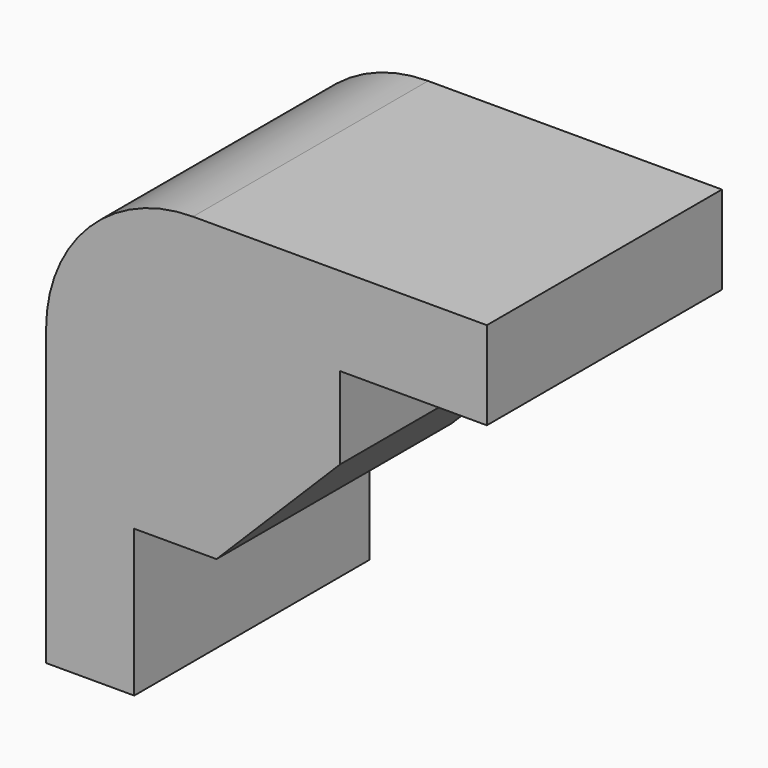
from build123d import *

# Parameters (mm, degrees)
F1_DEPTH = 12.7


# Not quite as in the source:
# - a feature names something its author has since deleted; it is built from what else it names


with BuildPart() as f1:
    # F0 (on Front) → F1 (new body)
    with BuildSketch(Plane.XZ):
        with BuildLine():
            Line((20.065747093, 21.1230388888), (20.065747093, 24.6790388888))
            Line((20.065747093, 24.6790388888), (26.415747093, 24.6790388888))
            Line((26.415747093, 24.6790388888), (26.415747093, 28.4890388888))
            Line((26.415747093, 28.4890388888), (13.715747093, 28.4890388888))
            ThreePointArc((13.715747093, 28.4890388888), (9.2256190324, 26.6291669493), (7.365747093, 22.1390388888))
            Line((7.365747093, 22.1390388888), (7.365747093, 9.4390388888))
            Line((7.365747093, 9.4390388888), (11.175747093, 9.4390388888))
            Line((11.175747093, 9.4390388888), (11.175747093, 15.7890388888))
            Line((11.175747093, 15.7890388888), (14.731747093, 15.7890388888))
            Line((14.731747093, 15.7890388888), (20.065747093, 21.1230388888))
        make_face()
    extrude(amount=F1_DEPTH)


solid = f1.part
